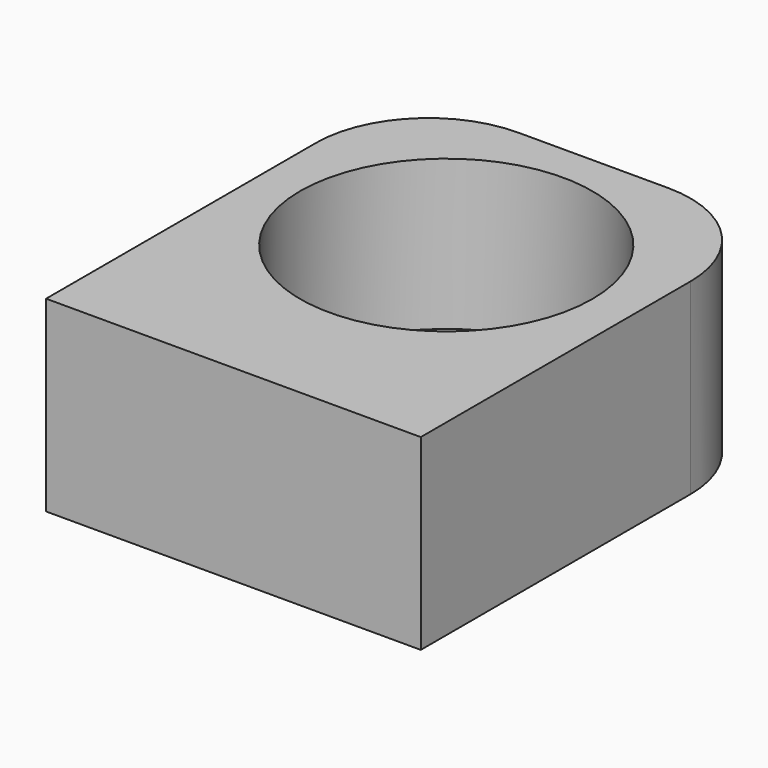
from build123d import *

# Parameters (mm, degrees)
F0_W     = 50
F0_H     = 60
F0_R     = 19.5
F1_DEPTH = 25
F2_R     = 15
F3_R     = 15
F4_R     = 19.5
F5_DEPTH = 5


with BuildPart() as f1:
    # F0 (on Top) → F1 (new body)
    with BuildSketch(Plane.XY):
        Rectangle(F0_W, F0_H)
        with Locations((0, 5.5)):
            Circle(F0_R, mode=Mode.SUBTRACT)
    extrude(amount=F1_DEPTH)

    # F2
    f2_edges = [f1.edges().sort_by_distance(p)[0] for p in [
        (-25, 30, 12.5),
    ]]
    fillet(f2_edges, radius=F2_R)

    # F3
    f3_edges = [f1.edges().sort_by_distance(p)[0] for p in [
        (25, 30, 12.5),
    ]]
    fillet(f3_edges, radius=F3_R)

    # F4 (on face) → F5 (join)
    with BuildSketch(Plane(origin=(0, 0, 0), x_dir=(1, 0, 0), z_dir=(0, 0, -1))):
        with Locations((0, -5.5)):
            Circle(F4_R)
    extrude(amount=-F5_DEPTH)


solid = f1.part
